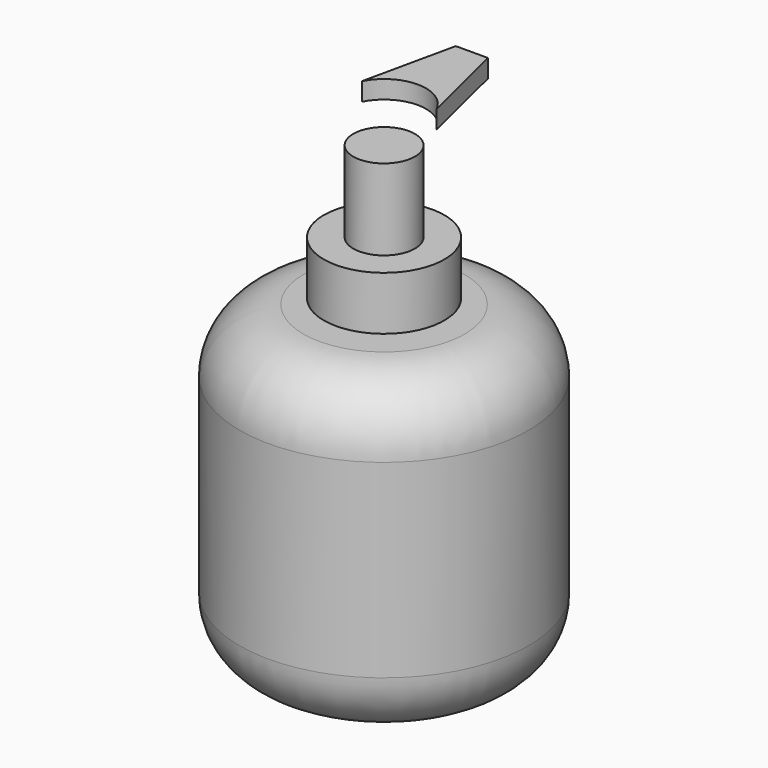
from build123d import *

# Parameters (mm, degrees)
F2_DEPTH = 13.462
F5_DEPTH = 8.636
F6_DEPTH = 4.318


# Not quite as in the source:
# - the program builds the solid bodies; features that only make, move or delete a surface that nothing else refers to are left out


with BuildPart() as f1:
    # F0 (on Front) → F1 (revolve)
    with BuildSketch(Plane.XZ):
        with BuildLine():
            Line((0, -75.8951976895), (0, -0.1828786626))
            Line((0, -0.1828786626), (-7.3489234783, -0.1828786626))
            Line((-7.3489234783, -0.1828786626), (-19.2328790224, -0.1828786626))
            ThreePointArc((-19.2328790224, -0.1828786626), (-30.0091863676, -4.6465713173), (-34.4728790224, -15.4228786626))
            Line((-34.4728790224, -15.4228786626), (-34.4728790224, -60.6551976895))
            ThreePointArc((-34.4728790224, -60.6551976895), (-30.0091863676, -71.4315050348), (-19.2328790224, -75.8951976895))
            Line((-19.2328790224, -75.8951976895), (0, -75.8951976895))
        make_face()
        Polygon((-7.3489234783, -0.1828786626), (0, -0.1828786626), (0, 0), (0, 19.7510421276), (-7.3489234783, 19.7510421276), (-7.3489234783, 13.8988820836), (-14.3560804427, 13.8988820836), (-14.3560804427, 1.0972818127), (-7.3489234783, 1.0972818127), align=None)
    revolve(axis=Axis((0, 0, 9.8755210638), (0, 0, -1)))

    # F2 (add): a face of the model
    f2_faces = [f1.faces().sort_by_distance(p)[0] for p in [
        (0, 0, 19.7510421276),
    ]]
    extrude(f2_faces, amount=F2_DEPTH)


with BuildPart() as f5:
    # F4 (on offset) → F5 (new body)
    with BuildSketch(Plane.XY.offset(33.274)):
        with BuildLine():
            ThreePointArc((-8.9320220688, 4.516127424), (0, 10.0088173701), (8.9320220688, 4.516127424))
            Line((8.9320220688, 4.516127424), (3.5661600996, 26.5176016837))
            Line((3.5661600996, 26.5176016837), (-4.1148001328, 26.5176016837))
            Line((-4.1148001328, 26.5176016837), (-8.9320220688, 4.516127424))
        make_face()
    extrude(amount=F5_DEPTH)

    # F6 (cut): a face of the model
    f6_faces = [f5.faces().sort_by_distance(p)[0] for p in [
        (-0.1584815304, 16.4759025541, 33.274),
    ]]
    extrude(f6_faces, amount=-F6_DEPTH, mode=Mode.SUBTRACT)


solid = Compound([f1.part, f5.part])
